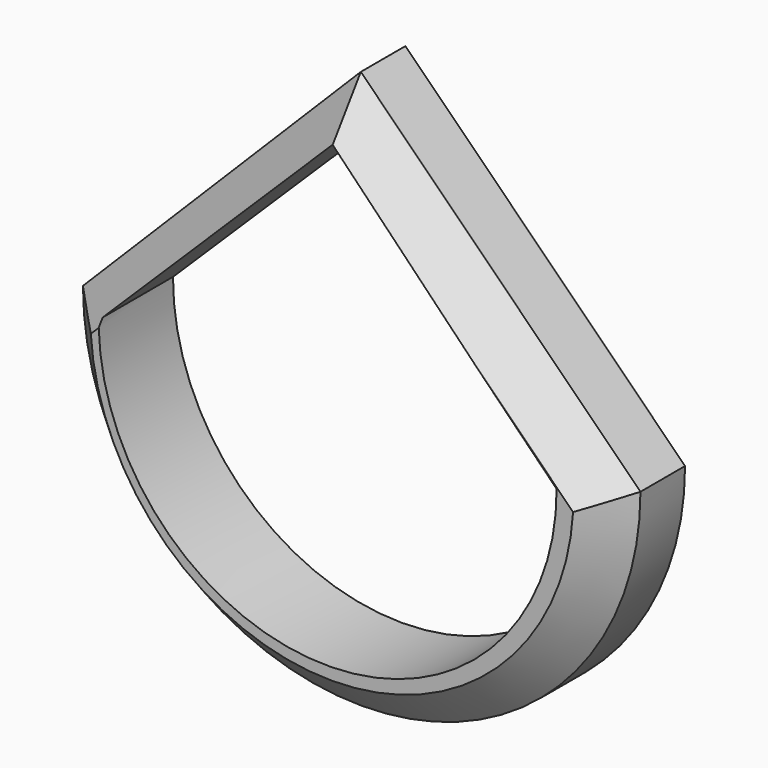
from build123d import *

# Parameters (mm, degrees)
F1_DEPTH    = 25.4
F3_DEPTH    = 25.4
F4_T1_DEPTH = 159.8348336794
F4_T3_DEPTH = 160.173130017
F4_T6_ANGLE = 219.4963428168


# Not quite as in the source:
# - a fillet or chamfer that OpenCascade refuses, or shapes differently, is made with other operations: its cross-section is extruded or revolved along the edge and cut away or added


with BuildPart() as f1:
    # F0 (on Front) → F1 (new body)
    with BuildSketch(Plane.XZ):
        with BuildLine():
            Line((76.4282107728, 0), (0, 76.1886239052))
            Line((0, 76.1886239052), (-75.9497880936, 0))
            ThreePointArc((-75.9497880936, 0), (0.2392113396, -76.2787980571), (76.4282107728, 0))
        make_face()
    extrude(amount=F1_DEPTH)

    # F2 (on Front) → F3 (cut)
    with BuildSketch(Plane.XZ):
        with BuildLine():
            Line((61.6340054605, 0), (0, 62.5749826431))
            Line((0, 62.5749826431), (-63.5303258896, 0))
            ThreePointArc((-63.5303258896, 0), (-0.9481602145, -62.9010402783), (61.6340054605, 0))
        make_face()
    extrude(amount=F3_DEPTH, mode=Mode.SUBTRACT)

    # F4: chamfer of 10.16 on 3 edges, made by hand

    # F4_s2 → F4_t1 (cut)
    with BuildSketch(Plane(origin=(56.5405950538, 0, 56.7183956672), x_dir=(0, 1, 0), z_dir=(-0.7059958535, 0, -0.7082159662))):
        Polygon((-15.24, -53.7888525608), (-25.4, -43.6288525608), (-25.4, -53.7888525608), align=None)
    extrude(amount=F4_T1_DEPTH, mode=Mode.SUBTRACT)

    # F4_s4 → F4_t3 (cut)
    with BuildSketch(Plane(origin=(56.8385652176, 0, -56.6603878972), x_dir=(0, 1, 0), z_dir=(-0.7082159662, 0, 0.7059958535))):
        Polygon((-15.24, -53.9579998959), (-25.4, -43.7979998959), (-25.4, -53.9579998959), align=None)
    extrude(amount=F4_T3_DEPTH, mode=Mode.SUBTRACT)

    # F4_s5 → F4_t6 (revolve, cut)
    with BuildSketch(Plane(origin=(-0.0012303148, 0, -0.0034270544), x_dir=(0, 1, 0), z_dir=(0.3378866803, 0, 0.9411867994))):
        Polygon((-15.24, 75.9335858363), (-25.4, 65.7735858363), (-25.4, 75.9335858363), align=None)
    revolve(axis=Axis((0.2392113396, -25.4, -0.0897457666), (0, -1, 0)), revolution_arc=F4_T6_ANGLE, mode=Mode.SUBTRACT)


solid = f1.part
